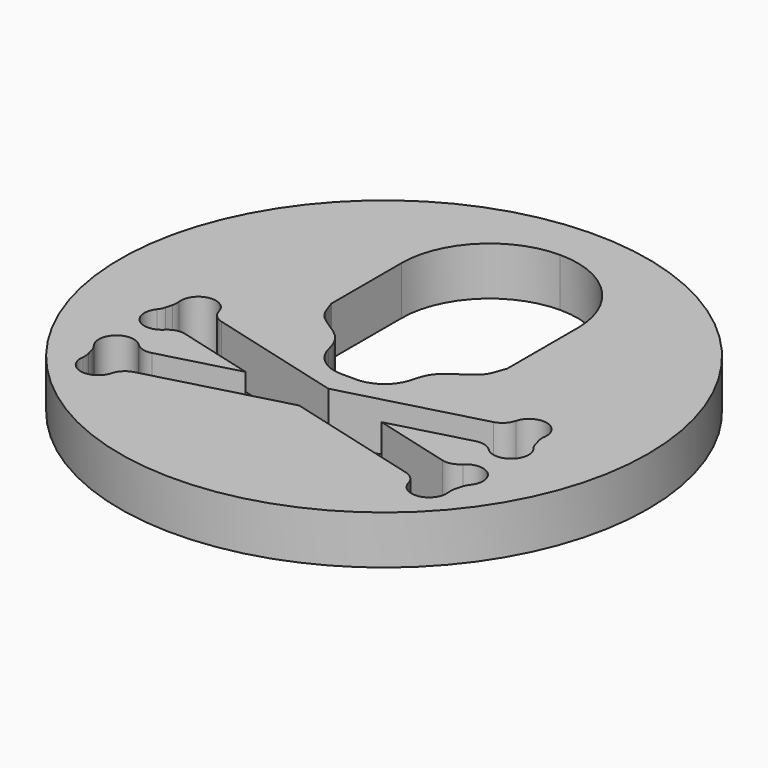
from build123d import *

# Parameters (mm, degrees)
F0_R     = 19.05
F1_DEPTH = 3.5
F3_DEPTH = 5.334
F5_DEPTH = 25.4


# Not quite as in the source:
# - a feature names something its author has since deleted; it is built from what else it names


with BuildPart() as f1:
    # F0 (on Top) → F1 (new body)
    with BuildSketch(Plane.XY):
        Circle(F0_R)
    extrude(amount=F1_DEPTH)

    # F2 (on face) → F3 (cut)
    with BuildSketch(Plane.XY.offset(3.5)):
        with BuildLine():
            Line((0, -3.175), (0.5430206191, -3.175))
            ThreePointArc((0.5430206191, -3.175), (2.1121063082, -2.6323908231), (3.0107980648, -1.2363937796))
            add(Edge.make_bspline(
                [(6.35, 3.175), (6.1354222845, 2.6541048515), (5.9660194487, 1.4359488031), (3.5744657813, 0.5479613391), (3.1233221277, -0.7746591325), (3.0107980648, -1.2363937796)],
                knots=[0, 0, 0, 0, 0.2694475223, 0.6162953248, 0.7809262502, 0.7809262502, 0.7809262502, 0.7809262502], degree=3))
            Line((6.35, 3.175), (6.35, 9.525))
            ThreePointArc((6.35, 9.525), (4.4901280605, 14.0151280605), (0, 15.875))
            Line((0, 15.875), (0, -3.175))
        make_face()
        with BuildLine():
            Line((-0.5430206191, -3.175), (0, -3.175))
            Line((0, -3.175), (0, 15.875))
            ThreePointArc((0, 15.875), (-4.4901280605, 14.0151280605), (-6.35, 9.525))
            Line((-6.35, 9.525), (-6.35, 3.175))
            add(Edge.make_bspline(
                [(-6.35, 3.175), (-6.1354222845, 2.6541048515), (-5.9660194487, 1.4359488031), (-3.5744657813, 0.5479613391), (-3.1233221277, -0.7746591325), (-3.0107980648, -1.2363937796)],
                knots=[0, 0, 0, 0, 0.2694475223, 0.6162953248, 0.7809262502, 0.7809262502, 0.7809262502, 0.7809262502], degree=3))
            ThreePointArc((-3.0107980648, -1.2363937796), (-2.1121063082, -2.6323908231), (-0.5430206191, -3.175))
        make_face()
    extrude(amount=-F3_DEPTH, mode=Mode.SUBTRACT)

    # F4 (on face) → F5 (cut)
    with BuildSketch(Plane.XY.offset(3.5)):
        with BuildLine():
            Line((-12.2672579939, -3.0629981272), (-11.9385578066, -1.8362723278))
            Line((-11.9385578066, -1.8362723278), (-9.8138063951, -2.4055977526))
            ThreePointArc((-9.8138063951, -2.4055977526), (-10.3831318199, -2.0768975654), (-10.7118320072, -1.5075721405))
            ThreePointArc((-10.7118320072, -1.5075721405), (-12.1993062273, -0.5933281371), (-13.1939593601, -2.0282799825))
            ThreePointArc((-13.1939593601, -2.0282799825), (-13.1812823619, -2.2901216321), (-13.2226351142, -2.5489878245))
            Line((-13.2226351142, -2.5489878245), (-13.3516440016, -3.030455547))
            ThreePointArc((-13.3516440016, -3.030455547), (-13.4452645639, -3.2753166219), (-13.5871639911, -3.4957396431))
            ThreePointArc((-13.5871639911, -3.4957396431), (-13.4432450328, -5.2357709608), (-11.697932569, -5.1877495387))
            ThreePointArc((-11.697932569, -5.1877495387), (-11.1286071442, -4.8590493514), (-10.4712067697, -4.8590493514))
            Line((-10.4712067697, -4.8590493514), (-12.5959581812, -4.2897239266))
            Line((-12.5959581812, -4.2897239266), (-12.2672579939, -3.0629981272))
        make_face()
        Polygon((-9.8138063951, -2.4055977526), (-11.9385578066, -1.8362723278), (-12.2672579939, -3.0629981272), (-2.4534515988, -5.6925996254), (0, -5.0351992509), align=None)
        Polygon((-2.4534515988, -5.6925996254), (-12.2672579939, -3.0629981272), (-12.5959581812, -4.2897239266), (-10.4712067697, -4.8590493514), (-4.9069031975, -6.35), align=None)
        with BuildLine():
            Line((9.8138063951, -2.4055977526), (0, -5.0351992509))
            Line((0, -5.0351992509), (2.4534515988, -5.6925996254))
            Line((2.4534515988, -5.6925996254), (4.9069031975, -6.35))
            Line((4.9069031975, -6.35), (10.4712067697, -4.8590493514))
            ThreePointArc((10.4712067697, -4.8590493514), (11.1286071442, -4.8590493514), (11.697932569, -5.1877495387))
            ThreePointArc((11.697932569, -5.1877495387), (13.4432450328, -5.2357709608), (13.5871639911, -3.4957396431))
            ThreePointArc((13.5871639911, -3.4957396431), (13.4452645639, -3.2753166219), (13.3516440016, -3.030455547))
            Line((13.3516440016, -3.030455547), (13.2226351142, -2.5489878245))
            ThreePointArc((13.2226351142, -2.5489878245), (13.1812823619, -2.2901216321), (13.1939593601, -2.0282799825))
            ThreePointArc((13.1939593601, -2.0282799825), (12.1993062273, -0.5933281371), (10.7118320072, -1.5075721405))
            ThreePointArc((10.7118320072, -1.5075721405), (10.3831318199, -2.0768975654), (9.8138063951, -2.4055977526))
        make_face()
        Polygon((0, -6.35), (0, -5.0351992509), (-2.4534515988, -5.6925996254), align=None)
        Polygon((2.4534515988, -5.6925996254), (0, -5.0351992509), (0, -6.35), align=None)
        Polygon((0, -6.35), (-2.4534515988, -5.6925996254), (-4.9069031975, -6.35), (-2.4534515988, -7.0074003746), align=None)
        Polygon((4.9069031975, -6.35), (2.4534515988, -5.6925996254), (0, -6.35), align=None)
        Polygon((4.9069031975, -6.35), (0, -6.35), (2.4534515988, -7.0074003746), align=None)
        Polygon((2.4534515988, -7.0074003746), (0, -6.35), (-2.4534515988, -7.0074003746), (0, -7.6648007491), align=None)
        Polygon((-2.4534515988, -7.0074003746), (-4.9069031975, -6.35), (-10.4712067697, -7.8409506486), (-12.5959581812, -8.4102760734), (-12.2672579939, -9.6370018728), align=None)
        Polygon((10.4712067697, -7.8409506486), (4.9069031975, -6.35), (2.4534515988, -7.0074003746), (12.2672579939, -9.6370018728), (12.5959581812, -8.4102760734), align=None)
        Polygon((12.2672579939, -9.6370018728), (2.4534515988, -7.0074003746), (0, -7.6648007491), (9.8138063951, -10.2944022474), (11.9385578066, -10.8637276722), align=None)
        Polygon((0, -7.6648007491), (-2.4534515988, -7.0074003746), (-12.2672579939, -9.6370018728), (-11.9385578066, -10.8637276722), (-9.8138063951, -10.2944022474), align=None)
        with BuildLine():
            Line((-12.5959581812, -8.4102760734), (-10.4712067697, -7.8409506486))
            ThreePointArc((-10.4712067697, -7.8409506486), (-11.1286071442, -7.8409506486), (-11.697932569, -7.5122504613))
            ThreePointArc((-11.697932569, -7.5122504613), (-13.4432450328, -7.4642290392), (-13.5871639911, -9.2042603569))
            ThreePointArc((-13.5871639911, -9.2042603569), (-13.4452645639, -9.4246833781), (-13.3516440016, -9.669544453))
            Line((-13.3516440016, -9.669544453), (-13.2226351142, -10.1510121755))
            ThreePointArc((-13.2226351142, -10.1510121755), (-13.1812823619, -10.4098783679), (-13.1939593601, -10.6717200175))
            ThreePointArc((-13.1939593601, -10.6717200175), (-12.1993062273, -12.1066718629), (-10.7118320072, -11.1924278595))
            ThreePointArc((-10.7118320072, -11.1924278595), (-10.3831318199, -10.6231024346), (-9.8138063951, -10.2944022474))
            Line((-9.8138063951, -10.2944022474), (-11.9385578066, -10.8637276722))
            Line((-11.9385578066, -10.8637276722), (-12.2672579939, -9.6370018728))
            Line((-12.2672579939, -9.6370018728), (-12.5959581812, -8.4102760734))
        make_face()
        with BuildLine():
            ThreePointArc((11.697932569, -7.5122504613), (11.1286071442, -7.8409506486), (10.4712067697, -7.8409506486))
            Line((10.4712067697, -7.8409506486), (12.5959581812, -8.4102760734))
            Line((12.5959581812, -8.4102760734), (12.2672579939, -9.6370018728))
            Line((12.2672579939, -9.6370018728), (11.9385578066, -10.8637276722))
            Line((11.9385578066, -10.8637276722), (9.8138063951, -10.2944022474))
            ThreePointArc((9.8138063951, -10.2944022474), (10.3831318199, -10.6231024346), (10.7118320072, -11.1924278595))
            ThreePointArc((10.7118320072, -11.1924278595), (12.1993062273, -12.1066718629), (13.1939593601, -10.6717200175))
            ThreePointArc((13.1939593601, -10.6717200175), (13.1812823619, -10.4098783679), (13.2226351142, -10.1510121755))
            Line((13.2226351142, -10.1510121755), (13.3516440016, -9.669544453))
            ThreePointArc((13.3516440016, -9.669544453), (13.4452645639, -9.4246833781), (13.5871639911, -9.2042603569))
            ThreePointArc((13.5871639911, -9.2042603569), (13.4432450328, -7.4642290392), (11.697932569, -7.5122504613))
        make_face()
    extrude(amount=-F5_DEPTH, mode=Mode.SUBTRACT)


solid = f1.part
